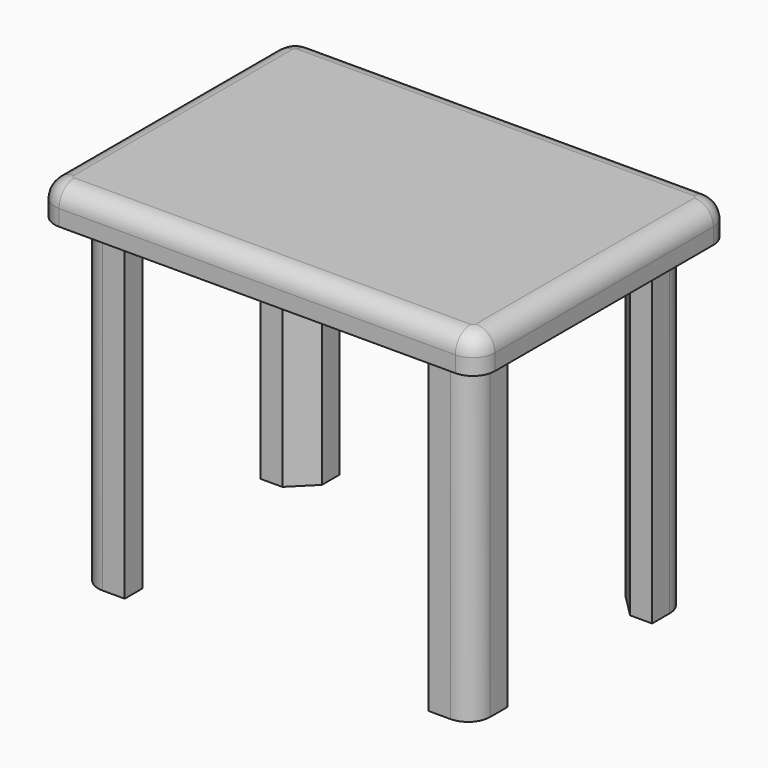
from build123d import *

# Parameters (mm, degrees)
F0_W         = 100
F0_H         = 72
F1_DEPTH     = 8
F2_T         = -2.5
F3_W         = 10
F3_H         = 10
F4_DEPTH     = 78.7
F5_R         = 4.3455844123
F6_R         = 5
F7_T1_DEPTH  = 20.5
F7_T3_DEPTH  = 91.2
F7_T6_ANGLE  = 90
F7_T8_ANGLE  = 90
F7_T10_ANGLE = 90
F8_SIZE      = 5
F9_T1_DEPTH  = 20.5
F9_T4_ANGLE  = 90


# Not quite as in the source:
# - a fillet or chamfer that OpenCascade refuses, or shapes differently, is made with other operations: its cross-section is extruded or revolved along the edge and cut away or added


with BuildPart() as f1:
    # F0 (on Top) → F1 (new body)
    with BuildSketch(Plane.XY):
        Rectangle(F0_W, F0_H)
    extrude(amount=F1_DEPTH)

    # F2
    f2_openings = [f1.faces().sort_by_distance(p)[0] for p in [
        (0, 0, 0),
    ]]
    offset(amount=F2_T, openings=f2_openings)

    # F3 (on face) → F4 (join)
    with BuildSketch(Plane(origin=(0, 0, 5.5), x_dir=(1, 0, 0), z_dir=(0, 0, -1))):
        with Locations((-39.5, -25.5)):
            Rectangle(F3_W, F3_H)
        with Locations((39.5, -25.5)):
            Rectangle(F3_W, F3_H)
        with Locations((39.5, 25.5)):
            Rectangle(F3_W, F3_H)
        with Locations((-39.5, 25.5)):
            Rectangle(F3_W, F3_H)
    extrude(amount=F4_DEPTH)

    # F5
    f5_edges = [f1.edges().sort_by_distance(p)[0] for p in [
        (-50, 0, 8),
        (0, -36, 8),
        (50, 0, 8),
        (0, 36, 8),
    ]]
    fillet(f5_edges, radius=F5_R)

    # F6
    f6_edges = [f1.edges().sort_by_distance(p)[0] for p in [
        (-44.5, -30.5, -33.85),
    ]]
    fillet(f6_edges, radius=F6_R)

    # F7: fillet of radius 5 on 6 edges, made by hand

    # F7_s2 → F7_t1 (cut)
    with BuildSketch(Plane.XY.offset(-12.5)):
        with BuildLine():
            ThreePointArc((-50, -31), (-48.5355339059, -34.5355339059), (-45, -36))
            Line((-45, -36), (-50, -36))
            Line((-50, -36), (-50, -31))
        make_face()
        with BuildLine():
            ThreePointArc((-45, 36), (-48.5355339059, 34.5355339059), (-50, 31))
            Line((-50, 31), (-50, 36))
            Line((-50, 36), (-45, 36))
        make_face()
        with BuildLine():
            ThreePointArc((45, 36), (48.5355339059, 34.5355339059), (50, 31))
            Line((50, 31), (50, 36))
            Line((50, 36), (45, 36))
        make_face()
    extrude(amount=F7_T1_DEPTH, mode=Mode.SUBTRACT)

    # F7_s4 → F7_t3 (cut)
    with BuildSketch(Plane.XY.offset(-85.7)):
        with BuildLine():
            ThreePointArc((39.5, -30.5), (43.0355339059, -29.0355339059), (44.5, -25.5))
            Line((44.5, -25.5), (44.5, -30.5))
            Line((44.5, -30.5), (39.5, -30.5))
        make_face()
        with BuildLine():
            ThreePointArc((44.5, 25.5), (43.0355339059, 29.0355339059), (39.5, 30.5))
            Line((39.5, 30.5), (44.5, 30.5))
            Line((44.5, 30.5), (44.5, 25.5))
        make_face()
        with BuildLine():
            ThreePointArc((-39.5, 30.5), (-43.0355339059, 29.0355339059), (-44.5, 25.5))
            Line((-44.5, 25.5), (-44.5, 30.5))
            Line((-44.5, 30.5), (-39.5, 30.5))
        make_face()
    extrude(amount=F7_T3_DEPTH, mode=Mode.SUBTRACT)

    # F7_s5 → F7_t6 (revolve, cut)
    with BuildSketch(Plane.XZ.offset(-31)):
        with BuildLine():
            ThreePointArc((45.6544155877, 8), (48.7272077939, 6.7272077939), (50, 3.6544155877))
            Line((50, 3.6544155877), (50, 8))
            Line((50, 8), (45.6544155877, 8))
        make_face()
    revolve(axis=Axis((45, 31, 8), (0, 0, 1)), revolution_arc=F7_T6_ANGLE, mode=Mode.SUBTRACT)

    # F7_s7 → F7_t8 (revolve, cut)
    with BuildSketch(Plane.YZ.offset(-45)):
        with BuildLine():
            ThreePointArc((31.6544155877, 8), (34.7272077939, 6.7272077939), (36, 3.6544155877))
            Line((36, 3.6544155877), (36, 8))
            Line((36, 8), (31.6544155877, 8))
        make_face()
    revolve(axis=Axis((-45, 31, 8), (0, 0, 1)), revolution_arc=F7_T8_ANGLE, mode=Mode.SUBTRACT)

    # F7_s9 → F7_t10 (revolve, cut)
    with BuildSketch(Plane.XZ.offset(31)):
        with BuildLine():
            ThreePointArc((-45.6544155877, 8), (-48.7272077939, 6.7272077939), (-50, 3.6544155877))
            Line((-50, 3.6544155877), (-50, 8))
            Line((-50, 8), (-45.6544155877, 8))
        make_face()
    revolve(axis=Axis((-45, -31, 8), (0, 0, 1)), revolution_arc=F7_T10_ANGLE, mode=Mode.SUBTRACT)

    # F8
    f8_edges = [f1.edges().sort_by_distance(p)[0] for p in [
        (-34.5, -20.5, -33.85),
        (-34.5, 20.5, -33.85),
        (34.5, 20.5, -33.85),
        (34.5, -20.5, -33.85),
    ]]
    chamfer(f8_edges, length=F8_SIZE)

    # F9: fillet of radius 5 on 1 edges, made by hand

    # F9_s2 → F9_t1 (cut)
    with BuildSketch(Plane.XY.offset(-12.5)):
        with BuildLine():
            ThreePointArc((50, -31), (48.5355339059, -34.5355339059), (45, -36))
            Line((45, -36), (50, -36))
            Line((50, -36), (50, -31))
        make_face()
    extrude(amount=F9_T1_DEPTH, mode=Mode.SUBTRACT)

    # F9_s3 → F9_t4 (revolve, cut)
    with BuildSketch(Plane.YZ.offset(45)):
        with BuildLine():
            ThreePointArc((-31.6544155877, 8), (-34.7272077939, 6.7272077939), (-36, 3.6544155877))
            Line((-36, 3.6544155877), (-36, 8))
            Line((-36, 8), (-31.6544155877, 8))
        make_face()
    revolve(axis=Axis((45, -31, 8), (0, 0, 1)), revolution_arc=F9_T4_ANGLE, mode=Mode.SUBTRACT)


solid = f1.part
